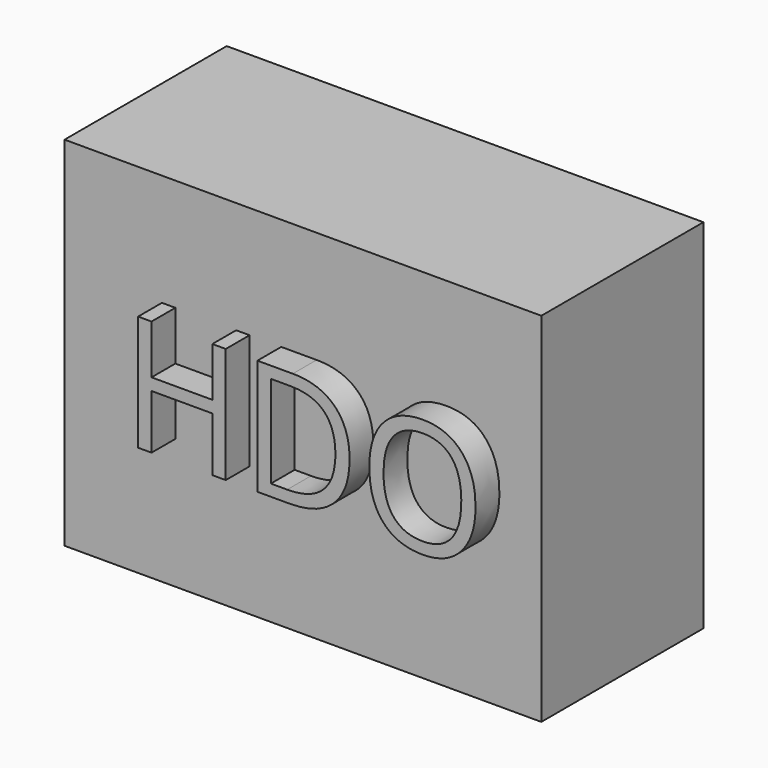
from build123d import *

# Parameters (mm, degrees)
F0_W         = 400
F0_H         = 300
F1_DEPTH     = 85
F2_TEXT_SIZE = 135.6799983316
F3_DEPTH     = 25


# Not quite as in the source:
# - Text() gives the source's letters only with a copy of the font that has no kerning and outlines rounded to 1/6400 em; it was checked with that copy


with BuildPart() as f1:
    # F0 (on Front) → F1 (new body, symmetric)
    with BuildSketch(Plane.XZ):
        Rectangle(F0_W, F0_H)
    extrude(amount=F1_DEPTH, both=True)

    # F2 (on face) → F3 (join)
    with BuildSketch(Plane.XZ.offset(85)):
        with Locations((-131.6304747015, -40.8292450011)):
            Text('HDO', F2_TEXT_SIZE, font='Open Sans', text_align=(TextAlign.LEFT, TextAlign.BOTTOM))
    extrude(amount=F3_DEPTH)


solid = f1.part
